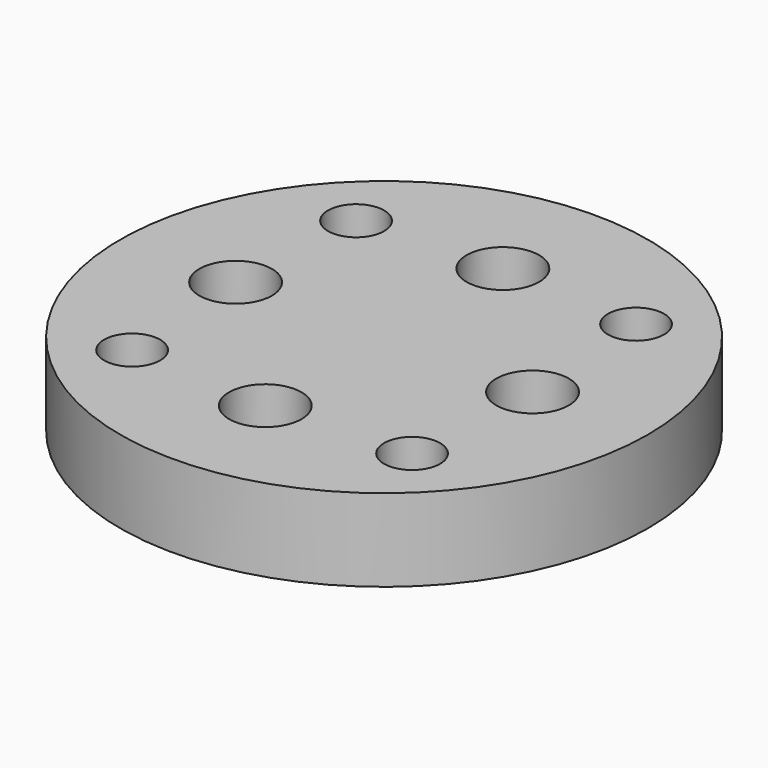
from build123d import *

# Parameters (mm, degrees)
F0_R                      = 8
F1_DEPTH                  = 2.5
F2_R                      = 1.1
F3_DEPTH                  = 2.501
F4_R                      = 0.85
F5_DEPTH                  = 2.501
F7_R                      = 1.75
F8_DEPTH                  = 0.5
F9_R                      = 1.75
F10_DEPTH                 = 25
DRAFT_F10_DRAFTED_ANGLE   = 45
DRAFT_F10_2_DRAFTED_ANGLE = 45
DRAFT_F10_3_DRAFTED_ANGLE = 45
DRAFT_F10_4_DRAFTED_ANGLE = 45


# Not quite as in the source:
# - an extrude with a draft is written as a straight extrude whose walls are then drafted


with BuildPart() as f1:
    # F0 (on Top) → F1 (new body)
    with BuildSketch(Plane.XY):
        Circle(F0_R)
    extrude(amount=F1_DEPTH)

    # F2 (on face) → F3 (cut, through all)
    with BuildSketch(Plane.XY.offset(2.5)):
        with Locations((0, 4.5)):
            Circle(F2_R)
        with Locations((-4.5, 0)):
            Circle(F2_R)
        with Locations((0, -4.5)):
            Circle(F2_R)
        with Locations((4.5, 0)):
            Circle(F2_R)
    extrude(amount=-F3_DEPTH, mode=Mode.SUBTRACT)

    # F4 (on face) → F5 (cut, through all)
    with BuildSketch(Plane(origin=(0, 0, 0), x_dir=(1, 0, 0), z_dir=(0, 0, -1))):
        with Locations((-4.2426406871, 4.2426406871)):
            Circle(F4_R)
        with Locations((4.2426406871, 4.2426406871)):
            Circle(F4_R)
        with Locations((4.2426406871, -4.2426406871)):
            Circle(F4_R)
        with Locations((-4.2426406871, -4.2426406871)):
            Circle(F4_R)
    extrude(amount=-F5_DEPTH, mode=Mode.SUBTRACT)

    # F7 (on Top) → F8 (cut)
    with BuildSketch(Plane.XY):
        with Locations((0, -4.5)):
            Circle(F7_R)
        with Locations((0, 4.5)):
            Circle(F7_R)
        with Locations((-4.5, 0)):
            Circle(F7_R)
        with Locations((4.5, 0)):
            Circle(F7_R)
    extrude(amount=F8_DEPTH, mode=Mode.SUBTRACT)


with BuildPart() as f10_drafted:
    # F9 (on face) → F10 (new body)
    with BuildSketch(Plane(origin=(0, 0, 0.5), x_dir=(1, 0, 0), z_dir=(0, 0, -1))):
        with Locations((0, 4.5)):
            Circle(F9_R)
    extrude(amount=-F10_DEPTH)

    # draft_F10_drafted
    draft_f10_drafted_walls = [f10_drafted.faces().sort_by_distance(p)[0] for p in [
        (-1.75, -4.5, 17.1666666667),
    ]]
    draft(draft_f10_drafted_walls, neutral_plane=Plane.XY.offset(0.5), angle=DRAFT_F10_DRAFTED_ANGLE)


with BuildPart() as f1_1:
    add(f1.part)

    # join_F10_drafted: cut F10_drafted
    add(f10_drafted.part, mode=Mode.SUBTRACT)


with BuildPart() as f10_2_drafted:
    # F9 (on face) → F10, piece 2 (new body)
    with BuildSketch(Plane(origin=(0, 0, 0.5), x_dir=(1, 0, 0), z_dir=(0, 0, -1))):
        with Locations((-4.5, 0)):
            Circle(F9_R)
    extrude(amount=-F10_DEPTH)

    # draft_F10_2_drafted
    draft_f10_2_drafted_walls = [f10_2_drafted.faces().sort_by_distance(p)[0] for p in [
        (-6.25, 0, 17.1666666667),
    ]]
    draft(draft_f10_2_drafted_walls, neutral_plane=Plane.XY.offset(0.5), angle=DRAFT_F10_2_DRAFTED_ANGLE)


with BuildPart() as f1_2:
    add(f1_1.part)

    # join_F10_2_drafted: cut F10_2_drafted
    add(f10_2_drafted.part, mode=Mode.SUBTRACT)


with BuildPart() as f10_3_drafted:
    # F9 (on face) → F10, piece 3 (new body)
    with BuildSketch(Plane(origin=(0, 0, 0.5), x_dir=(1, 0, 0), z_dir=(0, 0, -1))):
        with Locations((0, -4.5)):
            Circle(F9_R)
    extrude(amount=-F10_DEPTH)

    # draft_F10_3_drafted
    draft_f10_3_drafted_walls = [f10_3_drafted.faces().sort_by_distance(p)[0] for p in [
        (-1.75, 4.5, 17.1666666667),
    ]]
    draft(draft_f10_3_drafted_walls, neutral_plane=Plane.XY.offset(0.5), angle=DRAFT_F10_3_DRAFTED_ANGLE)


with BuildPart() as f1_3:
    add(f1_2.part)

    # join_F10_3_drafted: cut F10_3_drafted
    add(f10_3_drafted.part, mode=Mode.SUBTRACT)


with BuildPart() as f10_4_drafted:
    # F9 (on face) → F10, piece 4 (new body)
    with BuildSketch(Plane(origin=(0, 0, 0.5), x_dir=(1, 0, 0), z_dir=(0, 0, -1))):
        with Locations((4.5, 0)):
            Circle(F9_R)
    extrude(amount=-F10_DEPTH)

    # draft_F10_4_drafted
    draft_f10_4_drafted_walls = [f10_4_drafted.faces().sort_by_distance(p)[0] for p in [
        (2.75, 0, 17.1666666667),
    ]]
    draft(draft_f10_4_drafted_walls, neutral_plane=Plane.XY.offset(0.5), angle=DRAFT_F10_4_DRAFTED_ANGLE)


with BuildPart() as f1_4:
    add(f1_3.part)

    # join_F10_4_drafted: cut F10_4_drafted
    add(f10_4_drafted.part, mode=Mode.SUBTRACT)


solid = f1_4.part
